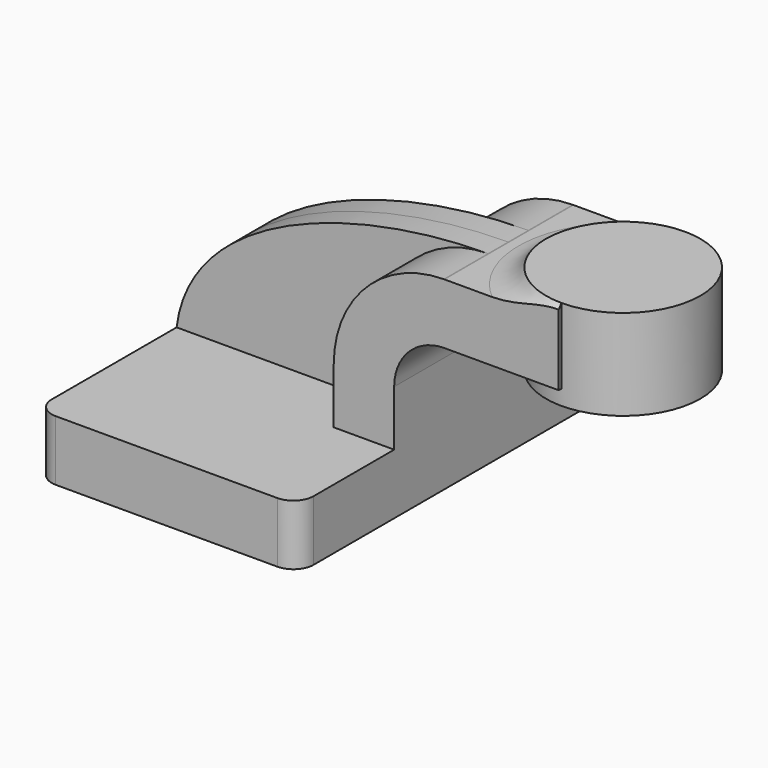
from build123d import *

# Parameters (mm, degrees)
F1_DEPTH    = 63.5
F0_W        = 26.465196414
F0_H        = 19.05
F2_DEPTH    = 25.4
F3_DEPTH    = 7.9375
F5_R        = 6.35
F6_T4_ANGLE = 180


# Not quite as in the source:
# - a fillet or chamfer that OpenCascade refuses, or shapes differently, is made with other operations: its cross-section is extruded or revolved along the edge and cut away or added


with BuildPart() as f1:
    # F0 (on Front) → F1 (new body, symmetric)
    with BuildSketch(Plane.XZ):
        Polygon((-41.275, -9.525), (41.275, -9.525), (41.275, 9.525), (22.225, 9.525), (-41.275, 9.525), align=None)
    extrude(amount=F1_DEPTH, both=True)

    # F0 (on Front) → F2 (join, symmetric)
    with BuildSketch(Plane.XZ):
        with BuildLine():
            Line((22.225, 9.525), (41.275, 9.525))
            Line((41.275, 9.525), (41.275, 27.0002))
            ThreePointArc((41.275, 27.0002), (45.9246798487, 38.2255201513), (57.15, 42.8752))
            Line((57.15, 42.8752), (66.675, 42.8752))
            Line((66.675, 42.8752), (66.675, 61.9252))
            Line((66.675, 61.9252), (57.15, 61.9252))
            add(Edge.make_bspline(
                [(56.9072220114, 61.9243561652), (56.9881728551, 61.9246965832), (57.0690989666, 61.9249778596), (57.15, 61.9252)],
                knots=[111.2968717992, 111.2968717992, 111.2968717992, 111.2968717992, 111.5045361635, 111.5045361635, 111.5045361635, 111.5045361635], degree=3))
            ThreePointArc((56.9072220114, 61.9243561652), (32.3686093383, 51.6099196626), (22.225, 27.0002))
            Line((22.225, 27.0002), (22.225, 9.525))
        make_face()
        with Locations((79.907598207, 52.4002)):
            Rectangle(F0_W, F0_H)
    extrude(amount=F2_DEPTH, both=True)

    # F0 (on Front) → F3 (join, symmetric)
    with BuildSketch(Plane.XZ):
        with BuildLine():
            add(Edge.make_bspline(
                [(-41.275, 9.525), (-36.9673291938, 44.5717190185), (13.5219464317, 61.7419104925), (56.9072220114, 61.9243561652)],
                knots=[0, 0, 0, 0, 111.2968717992, 111.2968717992, 111.2968717992, 111.2968717992], degree=3))
            Line((-41.275, 9.525), (22.225, 9.525))
            Line((22.225, 9.525), (22.225, 27.0002))
            ThreePointArc((22.225, 27.0002), (32.3686093383, 51.6099196626), (56.9072220114, 61.9243561652))
        make_face()
    extrude(amount=F3_DEPTH, both=True)

    # F0 (on Front) → F4 (revolve)
    with BuildSketch(Plane.XZ):
        Polygon((93.140196414, 61.9252), (93.140196414, 42.8752), (93.140196414, 38.1), (117.475, 38.1), (117.475, 66.675), (93.140196414, 66.675), align=None)
    revolve(axis=Axis((93.140196414, 0, 52.3875), (0, 0, -1)))

    # F5
    f5_edges = [f1.edges().sort_by_distance(p)[0] for p in [
        (-41.275, 63.5, 0),
        (-41.275, -63.5, 0),
        (41.275, -63.5, 0),
        (41.275, 63.5, 0),
    ]]
    fillet(f5_edges, radius=F5_R)

    # F6: fillet of radius 10.16 on 1 edges, made by hand


with BuildPart() as f6_tool2:
    # F6_s3 → F6_t4 (revolve)
    with BuildSketch(Plane.YZ.offset(93.140196414)):
        with BuildLine():
            ThreePointArc((32.9345324166, 61.9252), (28.0224061967, 63.1915721688), (24.334803586, 66.675))
            Line((24.334803586, 66.675), (24.334803586, 61.9252))
            Line((24.334803586, 61.9252), (32.9345324166, 61.9252))
        make_face()
    revolve(axis=Axis((93.140196414, 0, 61.9252), (0, 0, 1)), revolution_arc=F6_T4_ANGLE)

    split(bisect_by=Plane.XZ.offset(-25.4), keep=Keep.TOP)

    split(bisect_by=Plane.XZ.offset(25.4), keep=Keep.BOTTOM)


with BuildPart() as f1_1:
    add(f1.part)

    # F6_t1: union F6_tool2
    add(f6_tool2.part)


solid = f1_1.part
